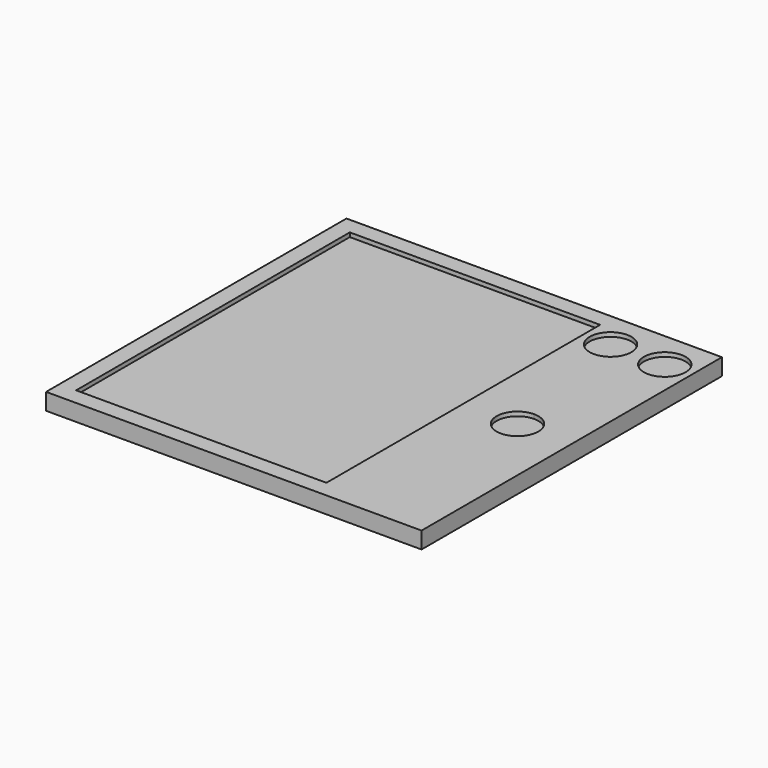
from build123d import *

# Parameters (mm, degrees)
F0_W      = 114.3
F0_H      = 114.3
F1_DEPTH  = 2.54
F8_W      = 114.3
F8_H      = 114.3
F9_DEPTH  = 2.54
F10_W     = 114.3
F10_H     = 114.3
F11_DEPTH = 2.54
F12_W     = 76.2
F12_H     = 104.14
F13_DEPTH = 1.27
F14_R     = 6.35
F15_DEPTH = 1.27
F17_W     = 111.252
F17_H     = 111.252
F18_DEPTH = 1.905


# Not quite as in the source:
# - a feature of the source that left no trace in its solid (it failed there, or was rolled back) is left out


with BuildPart() as f1:
    # F0 (on Top) → F1 (new body)
    with BuildSketch(Plane.XY):
        Rectangle(F0_W, F0_H)
    extrude(amount=F1_DEPTH)


with BuildPart() as f9:
    # F8 (on face) → F9 (new body)
    with BuildSketch(Plane.XY.offset(27.94)):
        Rectangle(F8_W, F8_H)
    extrude(amount=F9_DEPTH)

    # F10 (on face) → F11 (join)
    with BuildSketch(Plane.XY.offset(30.48)):
        Rectangle(F10_W, F10_H)
    extrude(amount=F11_DEPTH)

    # F12 (on face) → F13 (cut)
    with BuildSketch(Plane.XY.offset(33.02)):
        with Locations((-13.97, 0)):
            Rectangle(F12_W, F12_H)
    extrude(amount=-F13_DEPTH, mode=Mode.SUBTRACT)

    # F14 (on face) → F15 (cut)
    with BuildSketch(Plane.XY.offset(33.02)):
        with BuildLine():
            ThreePointArc((55.245, 45.72), (48.895, 52.07), (42.545, 45.72))
            ThreePointArc((42.545, 45.72), (48.895, 39.37), (55.245, 45.72))
        make_face()
        with Locations((32.385, 45.72)):
            Circle(F14_R)
        with BuildLine():
            ThreePointArc((40.64, 6.35), (36.1498719395, -4.4901280605), (46.99, 0))
            ThreePointArc((46.99, 0), (45.1301280605, 4.4901280605), (40.64, 6.35))
        make_face()
    extrude(amount=-F15_DEPTH, mode=Mode.SUBTRACT)


with BuildPart() as f18:
    # F17 (on face) → F18 (new body)
    with BuildSketch(Plane(origin=(0, 0, 27.94), x_dir=(1, 0, 0), z_dir=(0, 0, -1))):
        Rectangle(F17_W, F17_H)
    extrude(amount=F18_DEPTH)


solid = f9.part
